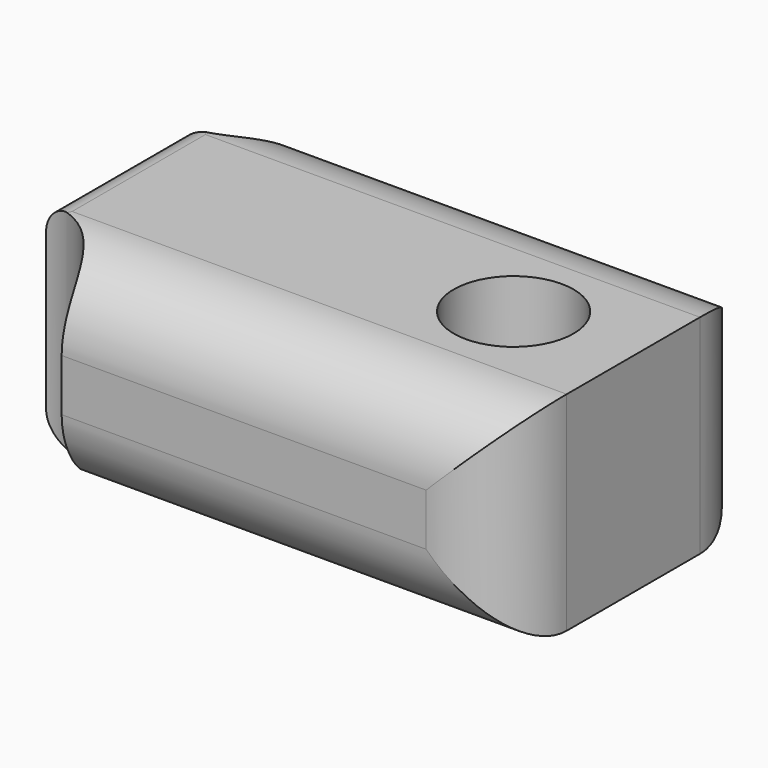
from build123d import *

# Parameters (mm, degrees)
F0_R        = 1.15
F1_DEPTH    = 4
F2_R        = 1.5
F3_DEPTH    = 5
F4_R        = 1.5
F5_T1_DEPTH = 5.7


# Not quite as in the source:
# - a fillet or chamfer that OpenCascade refuses, or shapes differently, is made with other operations: its cross-section is extruded or revolved along the edge and cut away or added


with BuildPart() as f1:
    # F0 (on Top) → F1 (new body)
    with BuildSketch(Plane.XY):
        with BuildLine():
            Line((5, 3.1), (-3.5, 3.1))
            ThreePointArc((-3.5, 3.1), (-3.93934, 2.03934), (-5, 1.6))
            Line((-5, 1.6), (-5, -1.6))
            ThreePointArc((-5, -1.6), (-3.93934, -2.03934), (-3.5, -3.1))
            Line((-3.5, -3.1), (5, -3.1))
            Line((5, -3.1), (5, 3.1))
        make_face()
        with Locations((2.7, 0)):
            Circle(F0_R, mode=Mode.SUBTRACT)
    extrude(amount=F1_DEPTH)

    # F2 (on face) → F3 (cut)
    with BuildSketch(Plane(origin=(-5, 0, 0), x_dir=(0, -1, 0), z_dir=(-1, 0, 0))):
        with Locations((0, 2)):
            Circle(F2_R)
    extrude(amount=-F3_DEPTH, mode=Mode.SUBTRACT)

    # F4
    f4_edges = [f1.edges().sort_by_distance(p)[0] for p in [
        (0.75, 3.1, 4),
        (0.75, 3.1, 0),
        (5, 3.1, 2),
        (5, -3.1, 2),
        (0.75, -3.1, 0),
        (0.75, -3.1, 4),
    ]]
    fillet(f4_edges, radius=F4_R)

    # F5: fillet of radius 0.5 on 2 edges, made by hand

    # F5_s2 → F5_t1 (cut)
    with BuildSketch(Plane.XZ.offset(-2.85)):
        with BuildLine():
            ThreePointArc((-5, 3.5), (-4.853553, 3.853553), (-4.5, 4))
            Line((-4.5, 4), (-5, 4))
            Line((-5, 4), (-5, 3.5))
        make_face()
        with BuildLine():
            ThreePointArc((-5, 0.5), (-4.853553, 0.146447), (-4.5, 0))
            Line((-4.5, 0), (-5, 0))
            Line((-5, 0), (-5, 0.5))
        make_face()
    extrude(amount=F5_T1_DEPTH, mode=Mode.SUBTRACT)


solid = f1.part
